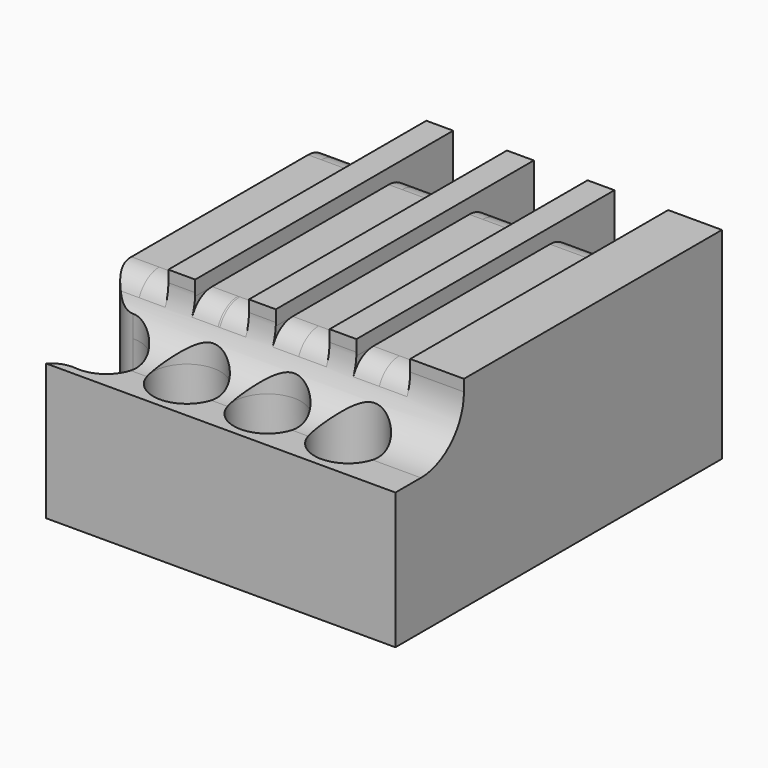
from build123d import *

# Parameters (mm, degrees)
F0_W         = 1
F0_H         = 3.475
F1_DEPTH     = 6
F2_DEPTH     = 1
F3_R         = 0.625
F4_DEPTH     = 0.66
F5_DEPTH     = 1.875
F6_T4_DEPTH  = 9
F6_S6_R      = 0.625
F6_T7_DEPTH  = 6
F6_T11_DEPTH = 9
F6_S14_R     = 0.625
F6_T15_DEPTH = 6
F6_S16_R     = 0.625
F6_T17_DEPTH = 6
F6_S18_R     = 0.625
F6_T19_DEPTH = 6
F6_S20_R     = 0.625
F6_T21_DEPTH = 6
F6_T25_DEPTH = 11.5
F6_T32_DEPTH = 11.5
F6_T39_DEPTH = 11.5
F7_T1_DEPTH  = 6.4537585313
F7_T3_DEPTH  = 4.9869031288
F7_T5_DEPTH  = 1
F7_T7_DEPTH  = 1
F7_T9_DEPTH  = 1
F7_T11_DEPTH = 2.25
F7_T13_DEPTH = 1.9833688147
F7_T18_DEPTH = 3.5
F7_T23_DEPTH = 3.5
F7_T28_DEPTH = 3.5
F7_T33_DEPTH = 3.5
F7_T38_DEPTH = 3.5
F7_T43_DEPTH = 3.5
F7_T48_DEPTH = 2.9667376294
F7_T53_DEPTH = 2.9667376294
F7_T58_DEPTH = 2.9667376294
F7_T63_DEPTH = 2.9667376294
F7_T68_DEPTH = 2.9667376294
F7_T73_DEPTH = 2.9667376294


# Not quite as in the source:
# - a fillet or chamfer that OpenCascade refuses, or shapes differently, is made with other operations: its cross-section is extruded or revolved along the edge and cut away or added


with BuildPart() as f1:
    # F0 (on Front) → F1 (new body)
    with BuildSketch(Plane.XZ):
        Polygon((2.25, -1.875), (3.25, -1.875), (3.25, 1.875), (2.25, 1.875), (2.25, 1.6), align=None)
        with Locations((1.75, -0.1375)):
            Rectangle(F0_W, F0_H)
        Polygon((0.75, -1.875), (1.25, -1.875), (1.25, 1.6), (1.25, 1.875), (0.75, 1.875), (0.75, 1.6), align=None)
        with Locations((0.25, -0.1375)):
            Rectangle(F0_W, F0_H)
        Polygon((-0.75, -1.875), (-0.25, -1.875), (-0.25, 1.6), (-0.25, 1.875), (-0.75, 1.875), (-0.75, 1.6), align=None)
        with Locations((-1.25, -0.1375)):
            Rectangle(F0_W, F0_H)
        Polygon((-2.25, -1.875), (-1.75, -1.875), (-1.75, 1.6), (-1.75, 1.875), (-2.25, 1.875), (-2.25, 1.6), align=None)
        with Locations((-2.75, -0.1375)):
            Rectangle(F0_W, F0_H)
    extrude(amount=F1_DEPTH)

    # F0 (on Front) → F2 (cut)
    with BuildSketch(Plane.XZ):
        with Locations((1.75, -0.1375)):
            Rectangle(F0_W, F0_H)
        with Locations((0.25, -0.1375)):
            Rectangle(F0_W, F0_H)
        with Locations((-1.25, -0.1375)):
            Rectangle(F0_W, F0_H)
        with Locations((-2.75, -0.1375)):
            Rectangle(F0_W, F0_H)
    extrude(amount=F2_DEPTH, mode=Mode.SUBTRACT)

    # F3 (on Top) → F4 (join, symmetric)
    with BuildSketch(Plane.XY):
        with BuildLine():
            Line((3.25, -6), (-3.25, -6))
            Line((-3.25, -6), (-3.25, -6.4440884776))
            ThreePointArc((-3.25, -6.4440884776), (-2.5523576462, -6.2261614164), (-2.125, -6.8190884776))
            ThreePointArc((-2.125, -6.8190884776), (-2.5523576462, -7.4120155389), (-3.25, -7.1940884776))
            Line((-3.25, -7.1940884776), (-3.25, -7.593262475))
            Line((-3.25, -7.593262475), (3.25, -7.593262475))
            Line((3.25, -7.593262475), (3.25, -6))
        make_face()
        with Locations((-1.25, -6.8190884776)):
            Circle(F3_R, mode=Mode.SUBTRACT)
        with Locations((0.25, -6.8190884776)):
            Circle(F3_R, mode=Mode.SUBTRACT)
        with Locations((1.75, -6.8190884776)):
            Circle(F3_R, mode=Mode.SUBTRACT)
    extrude(amount=F4_DEPTH, both=True)

    # F3 (on Top) → F5 (join)
    with BuildSketch(Plane.XY):
        with BuildLine():
            Line((3.25, -6), (-3.25, -6))
            Line((-3.25, -6), (-3.25, -6.4440884776))
            ThreePointArc((-3.25, -6.4440884776), (-2.5523576462, -6.2261614164), (-2.125, -6.8190884776))
            ThreePointArc((-2.125, -6.8190884776), (-2.5523576462, -7.4120155389), (-3.25, -7.1940884776))
            Line((-3.25, -7.1940884776), (-3.25, -7.593262475))
            Line((-3.25, -7.593262475), (3.25, -7.593262475))
            Line((3.25, -7.593262475), (3.25, -6))
        make_face()
        with Locations((-1.25, -6.8190884776)):
            Circle(F3_R, mode=Mode.SUBTRACT)
        with Locations((0.25, -6.8190884776)):
            Circle(F3_R, mode=Mode.SUBTRACT)
        with Locations((1.75, -6.8190884776)):
            Circle(F3_R, mode=Mode.SUBTRACT)
    extrude(amount=-F5_DEPTH)

    # F6: fillet of radius 1 on 1 edges, made by hand


with BuildPart() as f6_tool2:
    # F6_s3 → F6_t4 (new body)
    with BuildSketch(Plane.YZ.offset(3.25)):
        with BuildLine():
            ThreePointArc((-6, 1.66), (-6.2928932188, 0.9528932188), (-7, 0.66))
            Line((-7, 0.66), (-6, 0.66))
            Line((-6, 0.66), (-6, 1.66))
        make_face()
    extrude(amount=-F6_T4_DEPTH)

    split(bisect_by=Plane.YZ.offset(2.25), keep=Keep.TOP)

    # F6_s6 → F6_t7 (cut, symmetric)
    with BuildSketch(Plane.XY.offset(1.2)):
        with Locations((1.75, -6.8190884776)):
            Circle(F6_S6_R)
    extrude(amount=F6_T7_DEPTH, both=True, mode=Mode.SUBTRACT)


with BuildPart() as f1_1:
    add(f1.part)

    # F6_t1: union F6_tool2
    add(f6_tool2.part)


with BuildPart() as f6_tool9:
    # F6_s10 → F6_t11 (new body)
    with BuildSketch(Plane.YZ.offset(5.75)):
        with BuildLine():
            ThreePointArc((-6, 1.66), (-6.2928932188, 0.9528932188), (-7, 0.66))
            Line((-7, 0.66), (-6, 0.66))
            Line((-6, 0.66), (-6, 1.66))
        make_face()
    extrude(amount=-F6_T11_DEPTH)

    split(bisect_by=Plane.YZ.offset(2.25), keep=Keep.BOTTOM)

    split(bisect_by=Plane.XY.offset(1.6), keep=Keep.BOTTOM)

    # F6_s14 → F6_t15 (cut, symmetric)
    with BuildSketch(Plane.XY.offset(1.2)):
        with Locations((-2.75, -6.8190884776)):
            Circle(F6_S14_R)
    extrude(amount=F6_T15_DEPTH, both=True, mode=Mode.SUBTRACT)

    # F6_s16 → F6_t17 (cut, symmetric)
    with BuildSketch(Plane.XY.offset(1.2)):
        with Locations((1.75, -6.8190884776)):
            Circle(F6_S16_R)
    extrude(amount=F6_T17_DEPTH, both=True, mode=Mode.SUBTRACT)

    # F6_s18 → F6_t19 (cut, symmetric)
    with BuildSketch(Plane.XY.offset(1.2)):
        with Locations((0.25, -6.8190884776)):
            Circle(F6_S18_R)
    extrude(amount=F6_T19_DEPTH, both=True, mode=Mode.SUBTRACT)

    # F6_s20 → F6_t21 (cut, symmetric)
    with BuildSketch(Plane.XY.offset(1.2)):
        with Locations((-1.25, -6.8190884776)):
            Circle(F6_S20_R)
    extrude(amount=F6_T21_DEPTH, both=True, mode=Mode.SUBTRACT)


with BuildPart() as f1_2:
    add(f1_1.part)

    # F6_t8: union F6_tool9
    add(f6_tool9.part)


with BuildPart() as f6_tool23:
    # F6_s24 → F6_t25 (new body)
    with BuildSketch(Plane.YZ.offset(5.75)):
        with BuildLine():
            ThreePointArc((-6, 1.66), (-6.2928932188, 0.9528932188), (-7, 0.66))
            Line((-7, 0.66), (-6, 0.66))
            Line((-6, 0.66), (-6, 1.66))
        make_face()
    extrude(amount=-F6_T25_DEPTH)

    split(bisect_by=Plane.XY.offset(1.6), keep=Keep.TOP)

    split(bisect_by=Plane.YZ.offset(1.25), keep=Keep.BOTTOM)

    split(bisect_by=Plane.YZ.offset(0.75), keep=Keep.TOP)


with BuildPart() as f1_3:
    add(f1_2.part)

    # F6_t22: union F6_tool23
    add(f6_tool23.part)


with BuildPart() as f6_tool30:
    # F6_s31 → F6_t32 (new body)
    with BuildSketch(Plane.YZ.offset(5.75)):
        with BuildLine():
            ThreePointArc((-6, 1.66), (-6.2928932188, 0.9528932188), (-7, 0.66))
            Line((-7, 0.66), (-6, 0.66))
            Line((-6, 0.66), (-6, 1.66))
        make_face()
    extrude(amount=-F6_T32_DEPTH)

    split(bisect_by=Plane.XY.offset(1.6), keep=Keep.TOP)

    split(bisect_by=Plane.YZ.offset(-0.25), keep=Keep.BOTTOM)

    split(bisect_by=Plane.YZ.offset(-0.75), keep=Keep.TOP)


with BuildPart() as f1_4:
    add(f1_3.part)

    # F6_t29: union F6_tool30
    add(f6_tool30.part)


with BuildPart() as f6_tool37:
    # F6_s38 → F6_t39 (new body)
    with BuildSketch(Plane.YZ.offset(5.75)):
        with BuildLine():
            ThreePointArc((-6, 1.66), (-6.2928932188, 0.9528932188), (-7, 0.66))
            Line((-7, 0.66), (-6, 0.66))
            Line((-6, 0.66), (-6, 1.66))
        make_face()
    extrude(amount=-F6_T39_DEPTH)

    split(bisect_by=Plane.XY.offset(1.6), keep=Keep.TOP)

    split(bisect_by=Plane.YZ.offset(-1.75), keep=Keep.BOTTOM)

    split(bisect_by=Plane.YZ.offset(-2.25), keep=Keep.TOP)


with BuildPart() as f1_5:
    add(f1_4.part)

    # F6_t36: union F6_tool37
    add(f6_tool37.part)

    # F7: fillet of radius 0.5 on 10 edges, made by hand

    # F7_s2 → F7_t1 (cut)
    with BuildSketch(Plane.XY.offset(-3.75)):
        with BuildLine():
            ThreePointArc((-3.25, -5.6940884776), (-3.1035533906, -6.0476418682), (-2.75, -6.1940884776))
            ThreePointArc((-2.75, -6.1940884776), (-3.0295084972, -6.2600714833), (-3.25, -6.4440884776))
            Line((-3.25, -6.4440884776), (-3.25, -5.6940884776))
        make_face()
    extrude(amount=F7_T1_DEPTH, mode=Mode.SUBTRACT)

    # F7_s4 → F7_t3 (cut)
    with BuildSketch(Plane.XY.offset(-3.1009515644)):
        with BuildLine():
            ThreePointArc((-2.8254555009, -7.4395169323), (-3.0560709442, -7.4657378156), (-3.25, -7.593262475))
            Line((-3.25, -7.593262475), (-3.25, -7.1940884776))
            ThreePointArc((-3.25, -7.1940884776), (-3.0628035165, -7.3601790061), (-2.8254555009, -7.4395169323))
        make_face()
    extrude(amount=F7_T3_DEPTH, mode=Mode.SUBTRACT)

    # F7_s6 → F7_t5 (cut)
    with BuildSketch(Plane.YZ.offset(1.25)):
        with BuildLine():
            ThreePointArc((-1, 1.1), (-1.1464466094, 1.4535533906), (-1.5, 1.6))
            Line((-1.5, 1.6), (-1, 1.6))
            Line((-1, 1.6), (-1, 1.1))
        make_face()
        with BuildLine():
            ThreePointArc((-6.0723027314, 1.2866666667), (-5.8883350241, 1.5143267632), (-5.608454097, 1.6))
            Line((-5.608454097, 1.6), (-6.0018016229, 1.6))
            ThreePointArc((-6.0018016229, 1.6), (-6.024390983, 1.4404845199), (-6.0723027314, 1.2866666667))
        make_face()
    extrude(amount=F7_T5_DEPTH, mode=Mode.SUBTRACT)

    # F7_s8 → F7_t7 (cut)
    with BuildSketch(Plane.YZ.offset(-0.25)):
        with BuildLine():
            ThreePointArc((-1, 1.1), (-1.1464466094, 1.4535533906), (-1.5, 1.6))
            Line((-1.5, 1.6), (-1, 1.6))
            Line((-1, 1.6), (-1, 1.1))
        make_face()
        with BuildLine():
            ThreePointArc((-6.0723027314, 1.2866666667), (-5.8883350241, 1.5143267632), (-5.608454097, 1.6))
            Line((-5.608454097, 1.6), (-6.0018016229, 1.6))
            ThreePointArc((-6.0018016229, 1.6), (-6.024390983, 1.4404845199), (-6.0723027314, 1.2866666667))
        make_face()
    extrude(amount=F7_T7_DEPTH, mode=Mode.SUBTRACT)

    # F7_s10 → F7_t9 (cut)
    with BuildSketch(Plane.YZ.offset(-1.75)):
        with BuildLine():
            ThreePointArc((-1, 1.1), (-1.1464466094, 1.4535533906), (-1.5, 1.6))
            Line((-1.5, 1.6), (-1, 1.6))
            Line((-1, 1.6), (-1, 1.1))
        make_face()
        with BuildLine():
            ThreePointArc((-6.0723027314, 1.2866666667), (-5.8883350241, 1.5143267632), (-5.608454097, 1.6))
            Line((-5.608454097, 1.6), (-6.0018016229, 1.6))
            ThreePointArc((-6.0018016229, 1.6), (-6.024390983, 1.4404845199), (-6.0723027314, 1.2866666667))
        make_face()
    extrude(amount=F7_T9_DEPTH, mode=Mode.SUBTRACT)

    # F7_s12 → F7_t11 (cut)
    with BuildSketch(Plane.YZ.offset(-4.5)):
        with BuildLine():
            ThreePointArc((-1, 1.1), (-1.1464466094, 1.4535533906), (-1.5, 1.6))
            Line((-1.5, 1.6), (-1, 1.6))
            Line((-1, 1.6), (-1, 1.1))
        make_face()
    extrude(amount=F7_T11_DEPTH, mode=Mode.SUBTRACT)

    # F7_s14 → F7_t13 (cut)
    with BuildSketch(Plane.YZ.offset(-4.2333688147)):
        with BuildLine():
            ThreePointArc((-6.0723027314, 1.2866666667), (-5.8883350241, 1.5143267632), (-5.608454097, 1.6))
            Line((-5.608454097, 1.6), (-6.0018016229, 1.6))
            ThreePointArc((-6.0018016229, 1.6), (-6.024390983, 1.4404845199), (-6.0723027314, 1.2866666667))
        make_face()
    extrude(amount=F7_T13_DEPTH, mode=Mode.SUBTRACT)


with BuildPart() as f7_tool16:
    # F7_s17 → F7_t18 (new body)
    with BuildSketch(Plane.YZ.offset(3.5)):
        with BuildLine():
            ThreePointArc((-1, 1.1), (-1.1464466094, 1.4535533906), (-1.5, 1.6))
            Line((-1.5, 1.6), (-1, 1.6))
            Line((-1, 1.6), (-1, 1.1))
        make_face()
    extrude(amount=-F7_T18_DEPTH)

    split(bisect_by=Plane.YZ.offset(0.75), keep=Keep.BOTTOM)


with BuildPart() as f1_6:
    add(f1_5.part)

    # F7_t15: cut F7_tool16
    add(f7_tool16.part, mode=Mode.SUBTRACT)


with BuildPart() as f7_tool21:
    # F7_s22 → F7_t23 (new body)
    with BuildSketch(Plane.YZ.offset(2)):
        with BuildLine():
            ThreePointArc((-1, 1.1), (-1.1464466094, 1.4535533906), (-1.5, 1.6))
            Line((-1.5, 1.6), (-1, 1.6))
            Line((-1, 1.6), (-1, 1.1))
        make_face()
    extrude(amount=-F7_T23_DEPTH)

    split(bisect_by=Plane.YZ.offset(1.25), keep=Keep.TOP)


with BuildPart() as f1_7:
    add(f1_6.part)

    # F7_t20: cut F7_tool21
    add(f7_tool21.part, mode=Mode.SUBTRACT)


with BuildPart() as f7_tool26:
    # F7_s27 → F7_t28 (new body)
    with BuildSketch(Plane.YZ.offset(2)):
        with BuildLine():
            ThreePointArc((-1, 1.1), (-1.1464466094, 1.4535533906), (-1.5, 1.6))
            Line((-1.5, 1.6), (-1, 1.6))
            Line((-1, 1.6), (-1, 1.1))
        make_face()
    extrude(amount=-F7_T28_DEPTH)

    split(bisect_by=Plane.YZ.offset(-0.75), keep=Keep.BOTTOM)


with BuildPart() as f1_8:
    add(f1_7.part)

    # F7_t25: cut F7_tool26
    add(f7_tool26.part, mode=Mode.SUBTRACT)


with BuildPart() as f7_tool31:
    # F7_s32 → F7_t33 (new body)
    with BuildSketch(Plane.YZ.offset(0.5)):
        with BuildLine():
            ThreePointArc((-1, 1.1), (-1.1464466094, 1.4535533906), (-1.5, 1.6))
            Line((-1.5, 1.6), (-1, 1.6))
            Line((-1, 1.6), (-1, 1.1))
        make_face()
    extrude(amount=-F7_T33_DEPTH)

    split(bisect_by=Plane.YZ.offset(-0.25), keep=Keep.TOP)


with BuildPart() as f1_9:
    add(f1_8.part)

    # F7_t30: cut F7_tool31
    add(f7_tool31.part, mode=Mode.SUBTRACT)


with BuildPart() as f7_tool36:
    # F7_s37 → F7_t38 (new body)
    with BuildSketch(Plane.YZ.offset(0.5)):
        with BuildLine():
            ThreePointArc((-1, 1.1), (-1.1464466094, 1.4535533906), (-1.5, 1.6))
            Line((-1.5, 1.6), (-1, 1.6))
            Line((-1, 1.6), (-1, 1.1))
        make_face()
    extrude(amount=-F7_T38_DEPTH)

    split(bisect_by=Plane.YZ.offset(-2.25), keep=Keep.BOTTOM)


with BuildPart() as f1_10:
    add(f1_9.part)

    # F7_t35: cut F7_tool36
    add(f7_tool36.part, mode=Mode.SUBTRACT)


with BuildPart() as f7_tool41:
    # F7_s42 → F7_t43 (new body)
    with BuildSketch(Plane.YZ.offset(-1)):
        with BuildLine():
            ThreePointArc((-1, 1.1), (-1.1464466094, 1.4535533906), (-1.5, 1.6))
            Line((-1.5, 1.6), (-1, 1.6))
            Line((-1, 1.6), (-1, 1.1))
        make_face()
    extrude(amount=-F7_T43_DEPTH)

    split(bisect_by=Plane.YZ.offset(-1.75), keep=Keep.TOP)


with BuildPart() as f1_11:
    add(f1_10.part)

    # F7_t40: cut F7_tool41
    add(f7_tool41.part, mode=Mode.SUBTRACT)


with BuildPart() as f7_tool46:
    # F7_s47 → F7_t48 (new body)
    with BuildSketch(Plane.YZ.offset(0.2666311853)):
        with BuildLine():
            ThreePointArc((-6.0723027314, 1.2866666667), (-5.8883350241, 1.5143267632), (-5.608454097, 1.6))
            Line((-5.608454097, 1.6), (-6.0018016229, 1.6))
            ThreePointArc((-6.0018016229, 1.6), (-6.024390983, 1.4404845199), (-6.0723027314, 1.2866666667))
        make_face()
    extrude(amount=F7_T48_DEPTH)

    split(bisect_by=Plane.YZ.offset(0.75), keep=Keep.BOTTOM)


with BuildPart() as f1_12:
    add(f1_11.part)

    # F7_t45: cut F7_tool46
    add(f7_tool46.part, mode=Mode.SUBTRACT)


with BuildPart() as f7_tool51:
    # F7_s52 → F7_t53 (new body)
    with BuildSketch(Plane.YZ.offset(-1.2333688147)):
        with BuildLine():
            ThreePointArc((-6.0723027314, 1.2866666667), (-5.8883350241, 1.5143267632), (-5.608454097, 1.6))
            Line((-5.608454097, 1.6), (-6.0018016229, 1.6))
            ThreePointArc((-6.0018016229, 1.6), (-6.024390983, 1.4404845199), (-6.0723027314, 1.2866666667))
        make_face()
    extrude(amount=F7_T53_DEPTH)

    split(bisect_by=Plane.YZ.offset(-0.75), keep=Keep.BOTTOM)


with BuildPart() as f1_13:
    add(f1_12.part)

    # F7_t50: cut F7_tool51
    add(f7_tool51.part, mode=Mode.SUBTRACT)


with BuildPart() as f7_tool56:
    # F7_s57 → F7_t58 (new body)
    with BuildSketch(Plane.YZ.offset(-1.2333688147)):
        with BuildLine():
            ThreePointArc((-6.0723027314, 1.2866666667), (-5.8883350241, 1.5143267632), (-5.608454097, 1.6))
            Line((-5.608454097, 1.6), (-6.0018016229, 1.6))
            ThreePointArc((-6.0018016229, 1.6), (-6.024390983, 1.4404845199), (-6.0723027314, 1.2866666667))
        make_face()
    extrude(amount=F7_T58_DEPTH)

    split(bisect_by=Plane.YZ.offset(1.25), keep=Keep.TOP)


with BuildPart() as f1_14:
    add(f1_13.part)

    # F7_t55: cut F7_tool56
    add(f7_tool56.part, mode=Mode.SUBTRACT)


with BuildPart() as f7_tool61:
    # F7_s62 → F7_t63 (new body)
    with BuildSketch(Plane.YZ.offset(-2.7333688147)):
        with BuildLine():
            ThreePointArc((-6.0723027314, 1.2866666667), (-5.8883350241, 1.5143267632), (-5.608454097, 1.6))
            Line((-5.608454097, 1.6), (-6.0018016229, 1.6))
            ThreePointArc((-6.0018016229, 1.6), (-6.024390983, 1.4404845199), (-6.0723027314, 1.2866666667))
        make_face()
    extrude(amount=F7_T63_DEPTH)

    split(bisect_by=Plane.YZ.offset(-2.25), keep=Keep.BOTTOM)


with BuildPart() as f1_15:
    add(f1_14.part)

    # F7_t60: cut F7_tool61
    add(f7_tool61.part, mode=Mode.SUBTRACT)


with BuildPart() as f7_tool66:
    # F7_s67 → F7_t68 (new body)
    with BuildSketch(Plane.YZ.offset(-2.7333688147)):
        with BuildLine():
            ThreePointArc((-6.0723027314, 1.2866666667), (-5.8883350241, 1.5143267632), (-5.608454097, 1.6))
            Line((-5.608454097, 1.6), (-6.0018016229, 1.6))
            ThreePointArc((-6.0018016229, 1.6), (-6.024390983, 1.4404845199), (-6.0723027314, 1.2866666667))
        make_face()
    extrude(amount=F7_T68_DEPTH)

    split(bisect_by=Plane.YZ.offset(-0.25), keep=Keep.TOP)


with BuildPart() as f1_16:
    add(f1_15.part)

    # F7_t65: cut F7_tool66
    add(f7_tool66.part, mode=Mode.SUBTRACT)


with BuildPart() as f7_tool71:
    # F7_s72 → F7_t73 (new body)
    with BuildSketch(Plane.YZ.offset(-4.2333688147)):
        with BuildLine():
            ThreePointArc((-6.0723027314, 1.2866666667), (-5.8883350241, 1.5143267632), (-5.608454097, 1.6))
            Line((-5.608454097, 1.6), (-6.0018016229, 1.6))
            ThreePointArc((-6.0018016229, 1.6), (-6.024390983, 1.4404845199), (-6.0723027314, 1.2866666667))
        make_face()
    extrude(amount=F7_T73_DEPTH)

    split(bisect_by=Plane.YZ.offset(-1.75), keep=Keep.TOP)


with BuildPart() as f1_17:
    add(f1_16.part)

    # F7_t70: cut F7_tool71
    add(f7_tool71.part, mode=Mode.SUBTRACT)


solid = f1_17.part
